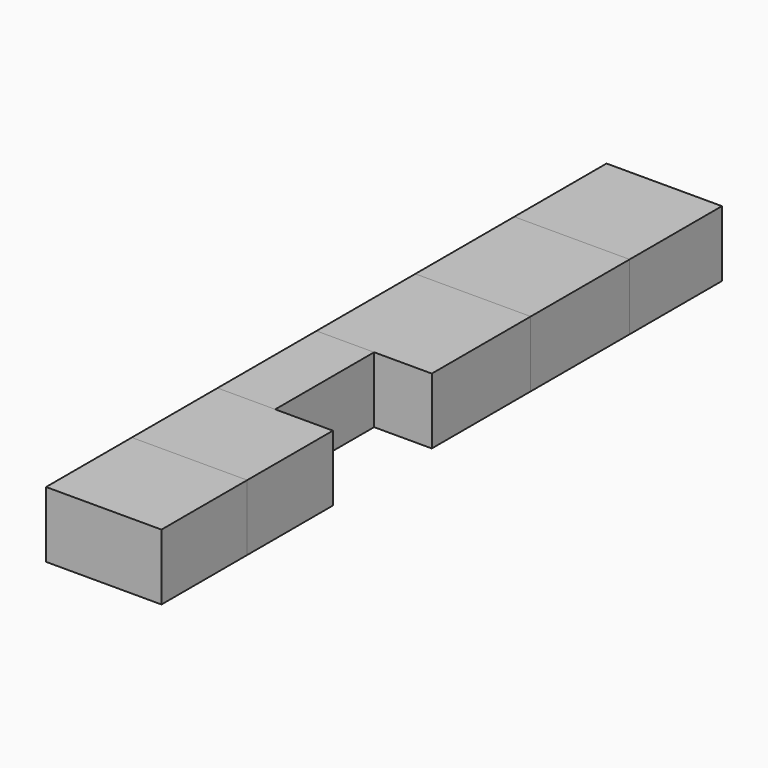
from build123d import *

# Parameters (mm, degrees)
F0_W     = 355.6
F0_H     = 660.4
F1_DEPTH = 406.4
F2_DEPTH = 406.4
F3_DEPTH = 406.4
F0_H_2   = 762
F4_DEPTH = 406.4
F5_DEPTH = 406.4
F0_H_3   = 711.2
F6_DEPTH = 406.4


# Not quite as in the source:
# - the program builds the solid bodies; features that only make, move or delete a surface that nothing else refers to are left out


with BuildPart() as f1:
    # F0 (on Top) → F1 (new body)
    with BuildSketch(Plane.XY):
        with Locations((-177.8, -1117.6)):
            Rectangle(F0_W, F0_H)
        with Locations((177.8, -1117.6)):
            Rectangle(F0_W, F0_H)
    extrude(amount=F1_DEPTH)


with BuildPart() as f2:
    # F0 (on Top) → F2 (new body)
    with BuildSketch(Plane.XY):
        with Locations((-177.8, -457.2)):
            Rectangle(F0_W, F0_H)
        with Locations((177.8, -457.2)):
            Rectangle(F0_W, F0_H)
    extrude(amount=F2_DEPTH)


with BuildPart() as f3:
    # F0 (on Top) → F3 (new body)
    with BuildSketch(Plane.XY):
        Polygon((0, 635), (-355.6, 635), (-355.6, 0), (-355.6, -127), (0, -127), align=None)
    extrude(amount=F3_DEPTH)


with BuildPart() as f4:
    # F0 (on Top) → F4 (new body)
    with BuildSketch(Plane.XY):
        with Locations((-177.8, 1016)):
            Rectangle(F0_W, F0_H_2)
        with Locations((177.8, 1016)):
            Rectangle(F0_W, F0_H_2)
    extrude(amount=F4_DEPTH)


with BuildPart() as f5:
    # F0 (on Top) → F5 (new body)
    with BuildSketch(Plane.XY):
        with Locations((-177.8, 1778)):
            Rectangle(F0_W, F0_H_2)
        with Locations((177.8, 1778)):
            Rectangle(F0_W, F0_H_2)
    extrude(amount=F5_DEPTH)


with BuildPart() as f6:
    # F0 (on Top) → F6 (new body)
    with BuildSketch(Plane.XY):
        with Locations((-177.8, 2514.6)):
            Rectangle(F0_W, F0_H_3)
        with Locations((177.8, 2514.6)):
            Rectangle(F0_W, F0_H_3)
    extrude(amount=F6_DEPTH)


solid = Compound([f1.part, f2.part, f3.part, f4.part, f5.part, f6.part])
